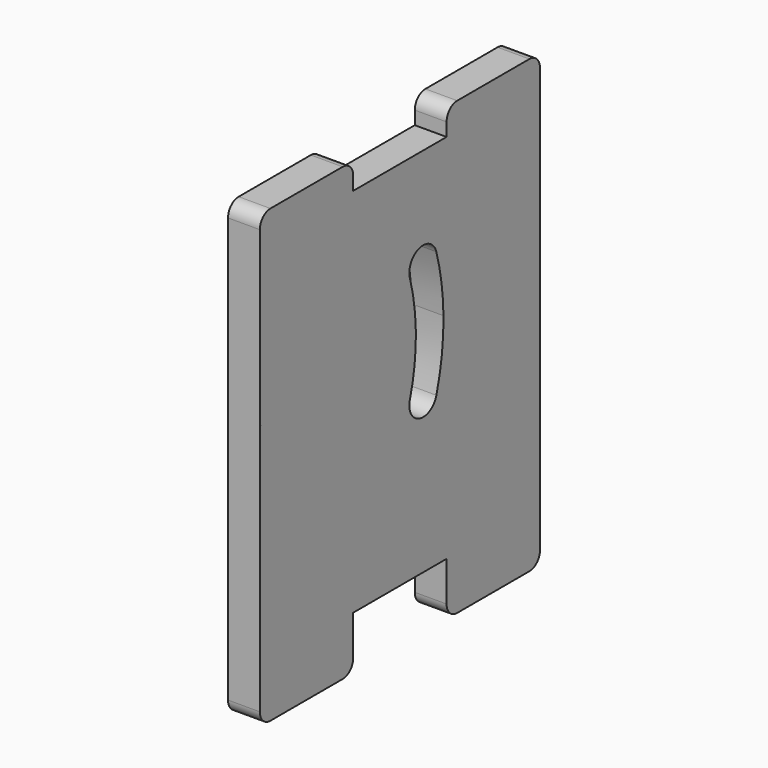
from build123d import *

# Parameters (mm, degrees)
F1_DEPTH = 3


# Not quite as in the source:
# - ends of sketch curves that miss each other by under 0.0002 mm in the source are joined


with BuildPart() as f1:
    # F0 (on Right) → F1 (new body)
    with BuildSketch(Plane.YZ):
        Polygon((5.5, 17.5), (-5.5, 17.5), (-16.5, 17.5), (-16.5, -17.5), (-5.5, -17.5), (5.5, -17.5), (16.5, -17.5), (16.5, 17.5), align=None)
        with BuildLine():
            Line((-16.4417464987, 2.5009048043), (-16.4935827024, 2.5))
            Line((-16.4935827024, 2.5), (-16.4660868868, 2.5078842983))
            Line((-16.4660868868, 2.5078842983), (1.1696009604, 7.5648364131))
            ThreePointArc((1.1696009604, 7.5648364131), (2.2837405131, 9.5747973722), (4.2937014722, 8.4606578195))
            ThreePointArc((4.2937014722, 8.4606578195), (4.8975775667, 5.6682772997), (5.1283712007, 2.8206836482))
            ThreePointArc((5.1283712007, 2.8206836482), (4.9431713186, -0.3431878735), (4.2978712002, -3.4460848682))
            ThreePointArc((4.2978712002, -3.4460848682), (2.2879051371, -4.5602229624), (1.1737655844, -2.5502620033))
            Line((1.1737655844, -2.5502620033), (-16.4417464987, 2.5009048043))
        make_face(mode=Mode.SUBTRACT)
        with BuildLine():
            Line((-5.5, -17.5), (-16.5, -17.5))
            Line((-16.5, -17.5), (-16.5, -21.2516473165))
            ThreePointArc((-16.5, -21.2516473165), (-16.1333008707, -22.1344656985), (-15.25, -22.5))
            Line((-15.25, -22.5), (-6.75, -22.5))
            ThreePointArc((-6.75, -22.5), (-5.8666991293, -22.1344656985), (-5.5000010855, -21.251647315))
            Line((-5.5000010855, -21.251647315), (-5.5, -17.5))
        make_face()
        with BuildLine():
            Line((16.5, -21.2516473165), (16.5, -17.5))
            Line((16.5, -17.5), (5.5, -17.5))
            Line((5.5, -17.5), (5.5, -21.251647316))
            ThreePointArc((5.5, -21.251647316), (5.8890966799, -22.1579284387), (6.8141527576, -22.5))
            Line((6.8141527576, -22.5), (15.3141527576, -22.5))
            ThreePointArc((15.3141527576, -22.5), (16.1562811226, -22.1125506362), (16.5, -21.2516473165))
        make_face()
        with BuildLine():
            Line((5.5, 18.75), (5.5, 17.5))
            Line((5.5, 17.5), (16.5, 17.5))
            Line((16.5, 17.5), (16.5, 18.75))
            ThreePointArc((16.5, 18.75), (16.1338834765, 19.6338834765), (15.25, 20))
            Line((15.25, 20), (6.75, 20))
            ThreePointArc((6.75, 20), (5.8661165235, 19.6338834765), (5.5, 18.75))
        make_face()
        with BuildLine():
            Line((-16.5, 17.5), (-5.5, 17.5))
            Line((-5.5, 17.5), (-5.5, 18.75))
            ThreePointArc((-5.5, 18.75), (-5.8661165235, 19.6338834765), (-6.75, 20))
            Line((-6.75, 20), (-15.25, 20))
            ThreePointArc((-15.25, 20), (-16.1338834765, 19.6338834765), (-16.5, 18.75))
            Line((-16.5, 18.75), (-16.5, 17.5))
        make_face()
        with BuildLine():
            Line((-16.4660868868, 2.5078842983), (-16.4417464987, 2.5009048043))
            Line((-16.4417464987, 2.5009048043), (1.8783712007, 2.8206836482))
            ThreePointArc((1.8783712007, 2.8206836482), (1.6794064974, 5.2159796384), (1.1696009604, 7.5648364131))
            Line((1.1696009604, 7.5648364131), (-16.4660868868, 2.5078842983))
        make_face()
        with BuildLine():
            Line((1.8783712007, 2.8206836482), (-16.4417464987, 2.5009048043))
            Line((-16.4417464987, 2.5009048043), (1.1737655844, -2.5502620033))
            ThreePointArc((1.1737655844, -2.5502620033), (1.7250108073, 0.1091116575), (1.8783712007, 2.8206836482))
        make_face()
    extrude(amount=F1_DEPTH)


solid = f1.part
